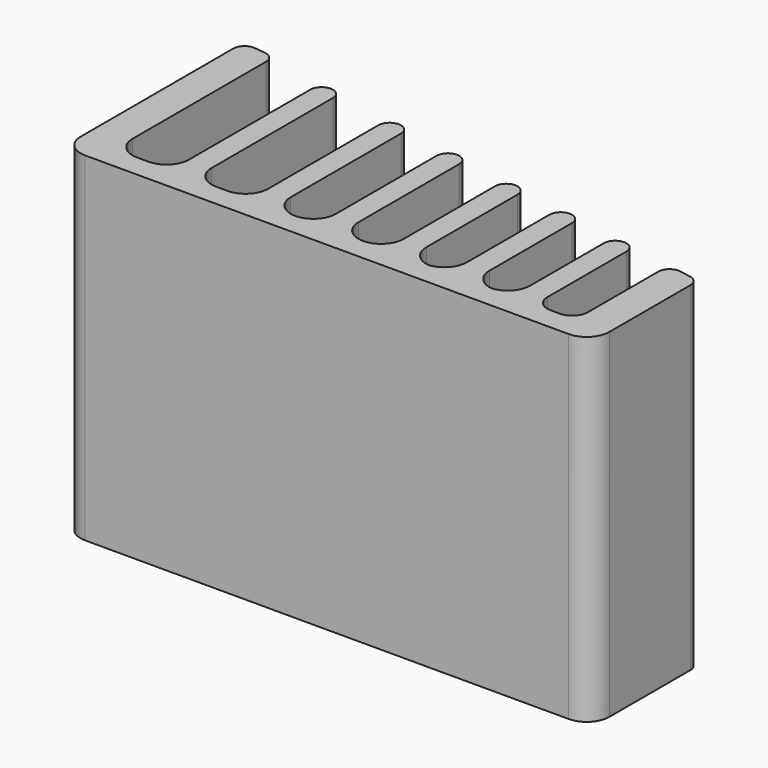
from build123d import *

# Parameters (mm, degrees)
F1_DEPTH    = 38.1
F2_T1_DEPTH = 38.1
F2_T3_DEPTH = 50.8
F3_T1_DEPTH = 38.1
F4_R        = 1.26999
F5_W        = 23.6700927116
F5_H        = 11.2887102096
F6_DEPTH    = 38.101
F7_R        = 2.54


# Not quite as in the source:
# - a fillet or chamfer that OpenCascade refuses, or shapes differently, is made with other operations: its cross-section is extruded or revolved along the edge and cut away or added
# - a fillet or chamfer is up to 0.001 mm smaller than in the source, because OpenCascade refuses the exact size


with BuildPart() as f1:
    # F0 (on Top) → F1 (new body)
    with BuildSketch(Plane.XY):
        Polygon((-36.3474, 25.4), (-36.3474, 0), (36.3474, 0), (36.3474, 12.7), (32.5374, 13.3656184486), (32.5374, 2.54), (29.337, 2.54), (29.337, 13.9247379455), (26.797, 14.3684835779), (26.797, 2.54), (23.0886, 2.54), (23.0886, 15.0163522013), (19.2786, 15.6819706499), (19.2786, 2.54), (14.7066, 2.54), (14.7066, 16.4807127883), (12.1666, 16.9244584207), (12.1666, 2.54), (7.5946, 2.54), (7.5946, 17.723200559), (5.0546, 18.1669461915), (5.0546, 2.54), (0.4826, 2.54), (0.4826, 18.9656883298), (-2.0574, 19.4094339623), (-2.0574, 2.54), (-7.1374, 2.54), (-7.1374, 20.2969252271), (-9.6774, 20.7406708595), (-9.6774, 2.54), (-14.7574, 2.54), (-14.7574, 21.6281621244), (-17.2974, 22.0719077568), (-17.2974, 2.54), (-23.6474, 2.54), (-23.6474, 23.1812718379), (-26.1874, 23.6250174703), (-26.1874, 2.54), (-32.5374, 2.54), (-32.5374, 24.9766666667), align=None)
    extrude(amount=F1_DEPTH)

    # F2: fillet of radius 2.54 on 14 edges, made by hand

    # F2_s2 → F2_t1 (join)
    with BuildSketch(Plane.XY):
        with BuildLine():
            ThreePointArc((-29.9974, 2.54), (-31.7934512242, 3.2839487758), (-32.5374, 5.08))
            Line((-32.5374, 5.08), (-32.5374, 2.54))
            Line((-32.5374, 2.54), (-29.9974, 2.54))
        make_face()
        with BuildLine():
            ThreePointArc((-26.1874, 5.08), (-26.9313487758, 3.2839487758), (-28.7274, 2.54))
            Line((-28.7274, 2.54), (-26.1874, 2.54))
            Line((-26.1874, 2.54), (-26.1874, 5.08))
        make_face()
        with BuildLine():
            ThreePointArc((-21.1074, 2.54), (-22.9034512242, 3.2839487758), (-23.6474, 5.08))
            Line((-23.6474, 5.08), (-23.6474, 2.54))
            Line((-23.6474, 2.54), (-21.1074, 2.54))
        make_face()
        with BuildLine():
            ThreePointArc((-17.2974, 5.08), (-18.0413487758, 3.2839487758), (-19.8374, 2.54))
            Line((-19.8374, 2.54), (-17.2974, 2.54))
            Line((-17.2974, 2.54), (-17.2974, 5.08))
        make_face()
        with BuildLine():
            ThreePointArc((-12.2174, 2.54), (-14.0134512242, 3.2839487758), (-14.7574, 5.08))
            Line((-14.7574, 5.08), (-14.7574, 2.54))
            Line((-14.7574, 2.54), (-12.2174, 2.54))
        make_face()
        with BuildLine():
            ThreePointArc((-9.6774, 5.08), (-10.4213487758, 3.2839487758), (-12.2174, 2.54))
            Line((-12.2174, 2.54), (-9.6774, 2.54))
            Line((-9.6774, 2.54), (-9.6774, 5.08))
        make_face()
        with BuildLine():
            ThreePointArc((-4.5974, 2.54), (-6.3934512242, 3.2839487758), (-7.1374, 5.08))
            Line((-7.1374, 5.08), (-7.1374, 2.54))
            Line((-7.1374, 2.54), (-4.5974, 2.54))
        make_face()
        with BuildLine():
            ThreePointArc((-2.0574, 5.08), (-2.8013487758, 3.2839487758), (-4.5974, 2.54))
            Line((-4.5974, 2.54), (-2.0574, 2.54))
            Line((-2.0574, 2.54), (-2.0574, 5.08))
        make_face()
        with BuildLine():
            ThreePointArc((3.0226, 2.54), (1.2265487758, 3.2839487758), (0.4826, 5.08))
            Line((0.4826, 5.08), (0.4826, 2.54))
            Line((0.4826, 2.54), (3.0226, 2.54))
        make_face()
        with BuildLine():
            ThreePointArc((5.0546, 5.08), (4.3106512242, 3.2839487758), (2.5146, 2.54))
            Line((2.5146, 2.54), (5.0546, 2.54))
            Line((5.0546, 2.54), (5.0546, 5.08))
        make_face()
        with BuildLine():
            ThreePointArc((10.1346, 2.54), (8.3385487758, 3.2839487758), (7.5946, 5.08))
            Line((7.5946, 5.08), (7.5946, 2.54))
            Line((7.5946, 2.54), (10.1346, 2.54))
        make_face()
        with BuildLine():
            ThreePointArc((12.1666, 5.08), (11.4226512242, 3.2839487758), (9.6266, 2.54))
            Line((9.6266, 2.54), (12.1666, 2.54))
            Line((12.1666, 2.54), (12.1666, 5.08))
        make_face()
    extrude(amount=F2_T1_DEPTH)

    # F2_s4 → F2_t3 (cut)
    with BuildSketch(Plane.XY.offset(-6.35)):
        with BuildLine():
            ThreePointArc((-33.8074, 0), (-35.6034512242, 0.7439487758), (-36.3474, 2.54))
            Line((-36.3474, 2.54), (-36.3474, 0))
            Line((-36.3474, 0), (-33.8074, 0))
        make_face()
        with BuildLine():
            ThreePointArc((36.3474, 2.54), (35.6034512242, 0.7439487758), (33.8074, 0))
            Line((33.8074, 0), (36.3474, 0))
            Line((36.3474, 0), (36.3474, 2.54))
        make_face()
    extrude(amount=F2_T3_DEPTH, mode=Mode.SUBTRACT)

    # F3: fillet of radius 1.778 on 6 edges, made by hand

    # F3_s2 → F3_t1 (join)
    with BuildSketch(Plane.XY):
        with BuildLine():
            ThreePointArc((14.7066, 4.318), (15.2273641431, 3.0607641431), (16.4846, 2.54))
            Line((16.4846, 2.54), (14.7066, 2.54))
            Line((14.7066, 2.54), (14.7066, 4.318))
        make_face()
        with BuildLine():
            ThreePointArc((17.5006, 2.54), (18.7578358569, 3.0607641431), (19.2786, 4.318))
            Line((19.2786, 4.318), (19.2786, 2.54))
            Line((19.2786, 2.54), (17.5006, 2.54))
        make_face()
        with BuildLine():
            ThreePointArc((23.0886, 4.318), (23.6093641431, 3.0607641431), (24.8666, 2.54))
            Line((24.8666, 2.54), (23.0886, 2.54))
            Line((23.0886, 2.54), (23.0886, 4.318))
        make_face()
        with BuildLine():
            ThreePointArc((25.019, 2.54), (26.2762358569, 3.0607641431), (26.797, 4.318))
            Line((26.797, 4.318), (26.797, 2.54))
            Line((26.797, 2.54), (25.019, 2.54))
        make_face()
        with BuildLine():
            ThreePointArc((29.337, 4.318), (29.8577641431, 3.0607641431), (31.115, 2.54))
            Line((31.115, 2.54), (29.337, 2.54))
            Line((29.337, 2.54), (29.337, 4.318))
        make_face()
        with BuildLine():
            ThreePointArc((30.7594, 2.54), (32.0166358569, 3.0607641431), (32.5374, 4.318))
            Line((32.5374, 4.318), (32.5374, 2.54))
            Line((32.5374, 2.54), (30.7594, 2.54))
        make_face()
    extrude(amount=F3_T1_DEPTH)

    # F4 (radius 1.27 in the source; OpenCascade refuses exactly that, so slightly less here)
    f4_edges = [f1.edges().sort_by_distance(p)[0] for p in [
        (32.5374, 13.365618, 19.05),
        (29.337, 13.924738, 19.05),
        (26.797, 14.368484, 19.05),
        (23.0886, 15.016352, 19.05),
        (19.2786, 15.681971, 19.05),
        (14.7066, 16.480713, 19.05),
        (12.1666, 16.924458, 19.05),
        (7.5946, 17.723201, 19.05),
        (5.0546, 18.166946, 19.05),
        (0.4826, 18.965688, 19.05),
        (-2.0574, 19.409434, 19.05),
        (-7.1374, 20.296925, 19.05),
        (-14.7574, 21.628162, 19.05),
        (-23.6474, 23.181272, 19.05),
        (-26.1874, 23.625017, 19.05),
        (-32.5374, 24.976667, 19.05),
        (-36.3474, 25.4, 19.05),
        (36.3474, 12.7, 19.05),
        (-9.6774, 20.740671, 19.05),
        (-17.2974, 22.071908, 19.05),
    ]]
    fillet(f4_edges, radius=F4_R)

    # F5 (on face) → F6 (cut, through all)
    with BuildSketch(Plane.XY.offset(38.1)):
        with Locations((34.9236463558, 19.5933448658)):
            Rectangle(F5_W, F5_H)
        Polygon((46.7586927116, 13.948989761), (23.0886, 13.948989761), (23.0886, -14.5505452529), (53.0812069774, -14.5505452529), (53.0812069774, 13.948989761), align=None)
    extrude(amount=-F6_DEPTH, mode=Mode.SUBTRACT)

    # F7
    f7_edges = [f1.edges().sort_by_distance(p)[0] for p in [
        (23.0886, 0, 19.05),
    ]]
    fillet(f7_edges, radius=F7_R)


solid = f1.part
